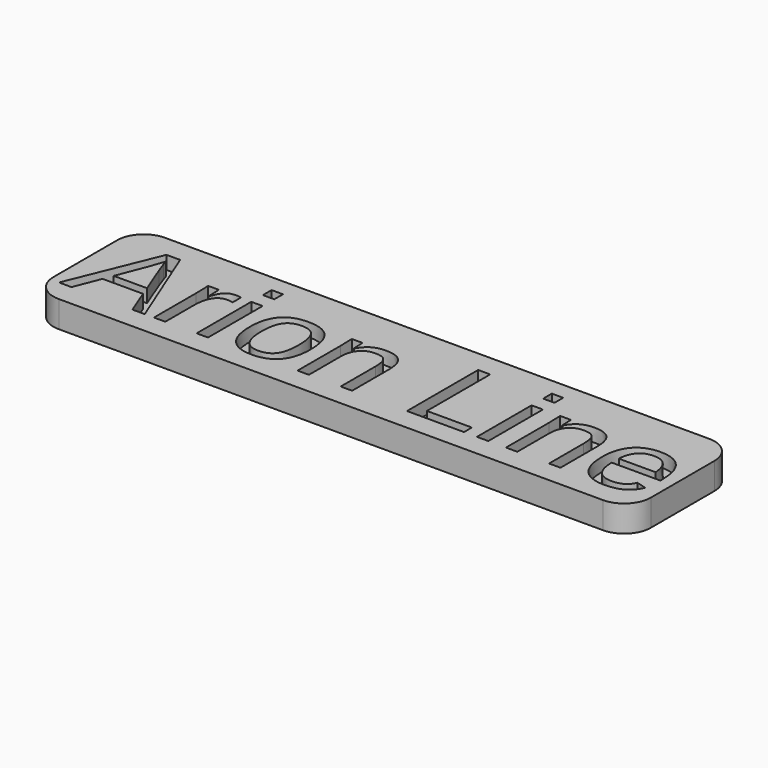
from build123d import *

# Parameters (mm, degrees)
F0_W         = 45
F0_H         = 10
F1_DEPTH     = 2
F2_TEXT_SIZE = 9.7374992846
F3_DEPTH     = 1
F4_R         = 2


# Not quite as in the source:
# - Text() gives the source's letters only with a copy of the font that has no kerning and outlines rounded to 1/6400 em; it was checked with that copy


with BuildPart() as f1:
    # F0 (on Top) → F1 (new body)
    with BuildSketch(Plane.XY):
        with Locations((22.5, 5)):
            Rectangle(F0_W, F0_H)
    extrude(amount=F1_DEPTH)

    # F2 (on face) → F3 (cut)
    with BuildSketch(Plane.XY.offset(2)):
        with Locations((0.6715932395, 1.6567144776)):
            Text('Arion Line', F2_TEXT_SIZE, font='Arimo', text_align=(TextAlign.LEFT, TextAlign.BOTTOM))
    extrude(amount=-F3_DEPTH, mode=Mode.SUBTRACT)

    # F4
    f4_edges = [f1.edges().sort_by_distance(p)[0] for p in [
        (0, 0, 1),
        (0, 10, 1),
        (45, 0, 1),
        (45, 10, 1),
    ]]
    fillet(f4_edges, radius=F4_R)


solid = f1.part
